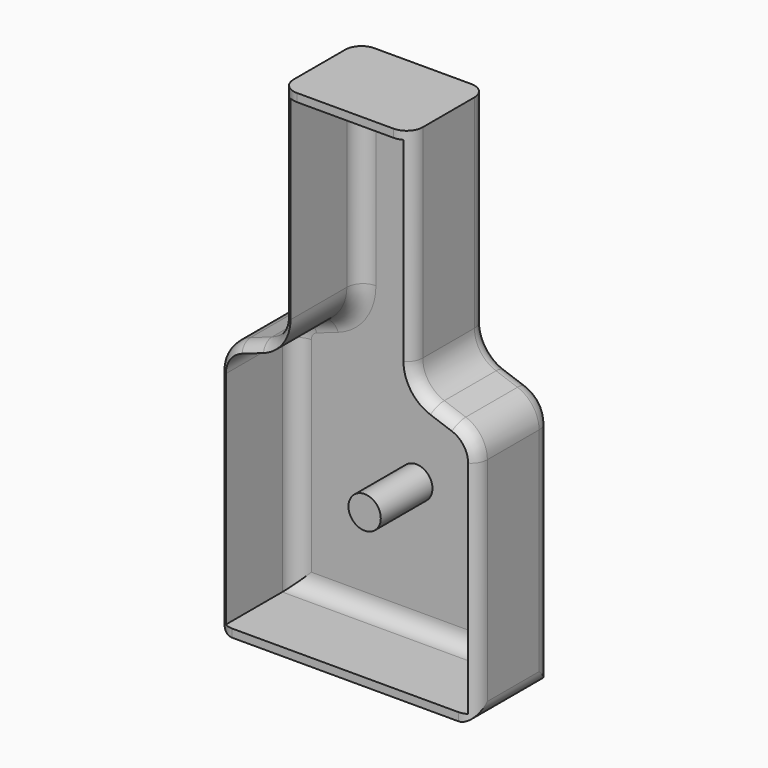
from build123d import *

# Parameters (mm, degrees)
F1_DEPTH     = 30
F2_T         = -2.5
F3_T1_DEPTH  = 55
F3_T3_DEPTH  = 83.3823547945
F3_T5_DEPTH  = 7.0343109423
F3_T7_DEPTH  = 75.4166657368
F3_T9_DEPTH  = 7.0343109423
F3_T12_ANGLE = 70.6224339747
F3_T14_ANGLE = 70.6224339747
F3_T16_ANGLE = 70.6224339747
F3_T18_ANGLE = 70.6224339747
F3_T20_ANGLE = 70.6224339747
F3_T22_ANGLE = 70.6224339747
F3_T24_ANGLE = 70.6224339747
F3_T26_ANGLE = 70.6224339747
F5_R         = 5
F6_DEPTH     = 20
F7_R         = 5


# Not quite as in the source:
# - a fillet or chamfer that OpenCascade refuses, or shapes differently, is made with other operations: its cross-section is extruded or revolved along the edge and cut away or added


with BuildPart() as f1:
    # F0 (on Front) → F1 (new body)
    with BuildSketch(Plane.XZ):
        with BuildLine():
            Line((20, 0), (0, 0))
            Line((0, 0), (-20, 0))
            Line((-20, 0), (-20, -62.9166657368))
            ThreePointArc((-20, -62.9166657368), (-21.8397555469, -68.6968396499), (-26.6820820931, -72.3501921592))
            Line((-26.6820820931, -72.3501921592), (-33.3179179069, -74.6841187831))
            ThreePointArc((-33.3179179069, -74.6841187831), (-38.1602444531, -78.3374712924), (-40, -84.1176452055))
            Line((-40, -84.1176452055), (-40, -155))
            Line((-40, -155), (0, -155))
            Line((0, -155), (40, -155))
            Line((40, -155), (40, -84.1176452055))
            ThreePointArc((40, -84.1176452055), (38.1602444531, -78.3374712924), (33.3179179069, -74.6841187831))
            Line((33.3179179069, -74.6841187831), (26.6820820931, -72.3501921592))
            ThreePointArc((26.6820820931, -72.3501921592), (21.8397555469, -68.6968396499), (20, -62.9166657368))
            Line((20, -62.9166657368), (20, 0))
        make_face()
    extrude(amount=F1_DEPTH)

    # F2
    f2_openings = [f1.faces().sort_by_distance(p)[0] for p in [
        (0, -30, -90.139239),
    ]]
    offset(amount=F2_T, openings=f2_openings)

    # F3: fillet of radius 5 on 8 edges, made by hand

    # F3_s2 → F3_t1 (cut)
    with BuildSketch(Plane.XZ.offset(-12.5)):
        with BuildLine():
            ThreePointArc((-35, -155), (-38.5355339059, -153.5355339059), (-40, -150))
            Line((-40, -150), (-40, -155))
            Line((-40, -155), (-35, -155))
        make_face()
        with BuildLine():
            ThreePointArc((40, -150), (38.5355339059, -153.5355339059), (35, -155))
            Line((35, -155), (40, -155))
            Line((40, -155), (40, -150))
        make_face()
    extrude(amount=F3_T1_DEPTH, mode=Mode.SUBTRACT)

    # F3_s4 → F3_t3 (cut)
    with BuildSketch(Plane.XY.offset(-167.5)):
        with BuildLine():
            ThreePointArc((-35, 0), (-38.5355339059, -1.4644660941), (-40, -5))
            Line((-40, -5), (-40, 0))
            Line((-40, 0), (-35, 0))
        make_face()
        with BuildLine():
            ThreePointArc((-40, -25), (-38.5355339059, -28.5355339059), (-35, -30))
            Line((-35, -30), (-40, -30))
            Line((-40, -30), (-40, -25))
        make_face()
        with BuildLine():
            ThreePointArc((35, 0), (38.5355339059, -1.4644660941), (40, -5))
            Line((40, -5), (40, 0))
            Line((40, 0), (35, 0))
        make_face()
        with BuildLine():
            ThreePointArc((40, -25), (38.5355339059, -28.5355339059), (35, -30))
            Line((35, -30), (40, -30))
            Line((40, -30), (40, -25))
        make_face()
    extrude(amount=F3_T3_DEPTH, mode=Mode.SUBTRACT)

    # F3_s6 → F3_t5 (cut)
    with BuildSketch(Plane(origin=(53.0259684291, 0, -18.6500574974), x_dir=(0, 1, 0), z_dir=(-0.9433526422, 0, 0.3317917907))):
        with BuildLine():
            ThreePointArc((-25, 59.3988491433), (-28.5355339059, 60.8633152374), (-30, 64.3988491433))
            Line((-30, 64.3988491433), (-30, 59.3988491433))
            Line((-30, 59.3988491433), (-25, 59.3988491433))
        make_face()
        with BuildLine():
            ThreePointArc((0, 64.3988491433), (-1.4644660941, 60.8633152374), (-5, 59.3988491433))
            Line((-5, 59.3988491433), (0, 59.3988491433))
            Line((0, 59.3988491433), (0, 64.3988491433))
        make_face()
    extrude(amount=F3_T5_DEPTH, mode=Mode.SUBTRACT)

    # F3_s8 → F3_t7 (cut)
    with BuildSketch(Plane.XY.offset(-62.9166657368)):
        with BuildLine():
            ThreePointArc((20, -25), (18.5355339059, -28.5355339059), (15, -30))
            Line((15, -30), (20, -30))
            Line((20, -30), (20, -25))
        make_face()
        with BuildLine():
            ThreePointArc((15, 0), (18.5355339059, -1.4644660941), (20, -5))
            Line((20, -5), (20, 0))
            Line((20, 0), (15, 0))
        make_face()
        with BuildLine():
            ThreePointArc((-20, -25), (-18.5355339059, -28.5355339059), (-15, -30))
            Line((-15, -30), (-20, -30))
            Line((-20, -30), (-20, -25))
        make_face()
        with BuildLine():
            ThreePointArc((-15, 0), (-18.5355339059, -1.4644660941), (-20, -5))
            Line((-20, -5), (-20, 0))
            Line((-20, 0), (-15, 0))
        make_face()
    extrude(amount=F3_T7_DEPTH, mode=Mode.SUBTRACT)

    # F3_s10 → F3_t9 (cut)
    with BuildSketch(Plane(origin=(-46.3901326153, 0, -16.3161308736), x_dir=(0, 1, 0), z_dir=(-0.9433526422, 0, -0.3317917907))):
        with BuildLine():
            ThreePointArc((-25, 59.3988491433), (-28.5355339059, 60.8633152374), (-30, 64.3988491433))
            Line((-30, 64.3988491433), (-30, 59.3988491433))
            Line((-30, 59.3988491433), (-25, 59.3988491433))
        make_face()
        with BuildLine():
            ThreePointArc((0, 64.3988491433), (-1.4644660941, 60.8633152374), (-5, 59.3988491433))
            Line((-5, 59.3988491433), (0, 59.3988491433))
            Line((0, 59.3988491433), (0, 64.3988491433))
        make_face()
    extrude(amount=F3_T9_DEPTH, mode=Mode.SUBTRACT)

    # F3_s11 → F3_t12 (revolve, cut)
    with BuildSketch(Plane.XY.offset(-84.1176452055)):
        with BuildLine():
            ThreePointArc((40, -25), (38.5355339059, -28.5355339059), (35, -30))
            Line((35, -30), (40, -30))
            Line((40, -30), (40, -25))
        make_face()
    revolve(axis=Axis((30, -30, -84.1176452055), (0, -1, 0)), revolution_arc=F3_T12_ANGLE, mode=Mode.SUBTRACT)

    # F3_s13 → F3_t14 (revolve, cut)
    with BuildSketch(Plane(origin=(46.3901326153, 0, -16.3161308736), x_dir=(0, 1, 0), z_dir=(0.9433526422, 0, -0.3317917907))):
        with BuildLine():
            ThreePointArc((-25, -59.3988491433), (-28.5355339059, -60.8633152374), (-30, -64.3988491433))
            Line((-30, -64.3988491433), (-30, -59.3988491433))
            Line((-30, -59.3988491433), (-25, -59.3988491433))
        make_face()
    revolve(axis=Axis((30, -30, -62.9166657368), (0, 1, 0)), revolution_arc=F3_T14_ANGLE, mode=Mode.SUBTRACT)

    # F3_s15 → F3_t16 (revolve, cut)
    with BuildSketch(Plane.XY.offset(-84.1176452055)):
        with BuildLine():
            ThreePointArc((35, 0), (38.5355339059, -1.4644660941), (40, -5))
            Line((40, -5), (40, 0))
            Line((40, 0), (35, 0))
        make_face()
    revolve(axis=Axis((30, 0, -84.1176452055), (0, -1, 0)), revolution_arc=F3_T16_ANGLE, mode=Mode.SUBTRACT)

    # F3_s17 → F3_t18 (revolve, cut)
    with BuildSketch(Plane(origin=(46.3901326153, 0, -16.3161308736), x_dir=(0, 1, 0), z_dir=(0.9433526422, 0, -0.3317917907))):
        with BuildLine():
            ThreePointArc((-5, -59.3988491433), (-1.4644660941, -60.8633152374), (0, -64.3988491433))
            Line((0, -64.3988491433), (0, -59.3988491433))
            Line((0, -59.3988491433), (-5, -59.3988491433))
        make_face()
    revolve(axis=Axis((30, 0, -62.9166657368), (0, 1, 0)), revolution_arc=F3_T18_ANGLE, mode=Mode.SUBTRACT)

    # F3_s19 → F3_t20 (revolve, cut)
    with BuildSketch(Plane(origin=(-53.0259684291, 0, -18.6500574974), x_dir=(0, 1, 0), z_dir=(0.9433526422, 0, 0.3317917907))):
        with BuildLine():
            ThreePointArc((-25, -59.3988491433), (-28.5355339059, -60.8633152374), (-30, -64.3988491433))
            Line((-30, -64.3988491433), (-30, -59.3988491433))
            Line((-30, -59.3988491433), (-25, -59.3988491433))
        make_face()
    revolve(axis=Axis((-30, -30, -84.1176452055), (0, -1, 0)), revolution_arc=F3_T20_ANGLE, mode=Mode.SUBTRACT)

    # F3_s21 → F3_t22 (revolve, cut)
    with BuildSketch(Plane.XY.offset(-62.9166657368)):
        with BuildLine():
            ThreePointArc((-20, -25), (-18.5355339059, -28.5355339059), (-15, -30))
            Line((-15, -30), (-20, -30))
            Line((-20, -30), (-20, -25))
        make_face()
    revolve(axis=Axis((-30, -30, -62.9166657368), (0, 1, 0)), revolution_arc=F3_T22_ANGLE, mode=Mode.SUBTRACT)

    # F3_s23 → F3_t24 (revolve, cut)
    with BuildSketch(Plane(origin=(-53.0259684291, 0, -18.6500574974), x_dir=(0, 1, 0), z_dir=(0.9433526422, 0, 0.3317917907))):
        with BuildLine():
            ThreePointArc((0, -64.3988491433), (-1.4644660941, -60.8633152374), (-5, -59.3988491433))
            Line((-5, -59.3988491433), (0, -59.3988491433))
            Line((0, -59.3988491433), (0, -64.3988491433))
        make_face()
    revolve(axis=Axis((-30, 0, -84.1176452055), (0, -1, 0)), revolution_arc=F3_T24_ANGLE, mode=Mode.SUBTRACT)

    # F3_s25 → F3_t26 (revolve, cut)
    with BuildSketch(Plane.XY.offset(-62.9166657368)):
        with BuildLine():
            ThreePointArc((-15, 0), (-18.5355339059, -1.4644660941), (-20, -5))
            Line((-20, -5), (-20, 0))
            Line((-20, 0), (-15, 0))
        make_face()
    revolve(axis=Axis((-30, 0, -62.9166657368), (0, 1, 0)), revolution_arc=F3_T26_ANGLE, mode=Mode.SUBTRACT)

    # F5 (on offset) → F6 (join)
    with BuildSketch(Plane.XZ.offset(22.5)):
        with Locations((0, -112.5)):
            Circle(F5_R)
    extrude(amount=-F6_DEPTH)

    # F7
    f7_edges = [f1.edges().sort_by_distance(p)[0] for p in [
        (-37.5, -2.5, -118.308823),
        (0, -2.5, -152.5),
        (0, -2.5, -2.5),
        (17.5, -2.5, -32.708333),
    ]]
    fillet(f7_edges, radius=F7_R)


solid = f1.part
